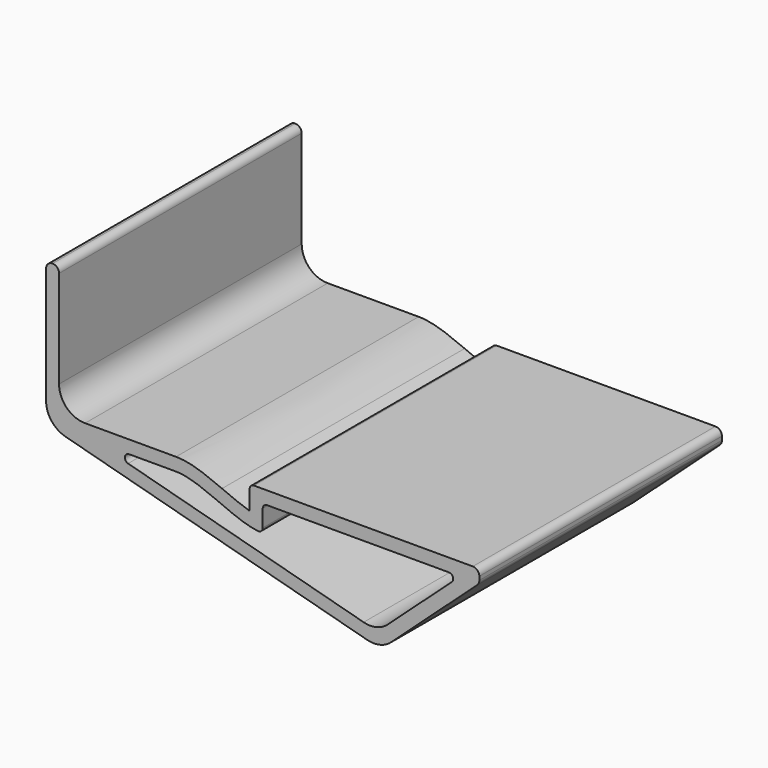
from build123d import *

# Parameters (mm, degrees)
F0_W         = 1.5
F0_H         = 15
F0_H_2       = 1.5
F1_DEPTH     = 35
F2_R         = 3
F3_R         = 0.5
F4_R         = 0.74999
F5_TEXT_SIZE = 7.8123211902
F6_DEPTH     = 0.4


# Not quite as in the source:
# - a fillet or chamfer is up to 0.001 mm smaller than in the source, because OpenCascade refuses the exact size
# - ends of sketch curves that miss each other by under 0.0002 mm in the source are joined
# - Text() gives the source's letters only with a copy of the font that has no kerning and outlines rounded to 1/6400 em; it was checked with that copy


with BuildPart() as f1:
    # F0 (on Front) → F1 (new body)
    with BuildSketch(Plane.XZ):
        with Locations((0.75, 9)):
            Rectangle(F0_W, F0_H)
        with BuildLine():
            Line((1.5, 1.5), (0, 1.5))
            Line((0, 1.5), (0, 0))
            Line((0, 0), (5.7955549577, 0))
            Line((5.7955549577, 0), (15, 0))
            Line((15, 0), (20.3076726165, 0))
            add(Edge.make_bspline(
                [(20.3076726165, 0), (19.9613391426, 0.1480763703), (19.1624921639, 0.4865686334), (17.8864112021, 0.9748848409), (16.4769611274, 1.3772161031), (15.5, 1.5), (15, 1.5)],
                knots=[0.5268596167, 0.5268596167, 0.5268596167, 0.5268596167, 0.625, 0.75, 0.875, 1, 1, 1, 1], degree=3))
            Line((15, 1.5), (1.5, 1.5))
        make_face()
        with BuildLine():
            add(Edge.make_bspline(
                [(23.5000271172, -1.2432669014), (23.3597225948, -1.2025116169), (22.8440957766, -1.0410149339), (21.8859439585, -0.6761057841), (20.9362434779, -0.2693177997), (20.4024591259, -0.0405263808), (20.3076726165, 0)],
                knots=[0.2014712136, 0.2014712136, 0.2014712136, 0.2014712136, 0.25, 0.375, 0.5, 0.5268596167, 0.5268596167, 0.5268596167, 0.5268596167], degree=3))
            Line((20.3076726165, 0), (15, 0))
            add(Edge.make_bspline(
                [(25, -3), (22, -3), (18, 0), (15, 0)],
                knots=[0, 0, 0, 0, 10.4403065089, 10.4403065089, 10.4403065089, 10.4403065089], degree=3))
            Line((25, -3), (25, 0))
            Line((25, 0), (23.5, 0))
            Line((23.5, 0), (23.5000271172, -1.2432669014))
        make_face()
        with Locations((24.25, 0.75)):
            Rectangle(F0_W, F0_H_2)
        Polygon((47.7727761903, 0), (50, 0), (50, 1.5), (25, 1.5), (25, 0), align=None)
        Polygon((39.0252616192, -8.9038730647), (38.6370330516, -10.3527618041), (50, 0), (47.7727761903, 0), (38.2330606413, -8.6916034524), align=None)
        Polygon((5.7955549577, 0), (0, 0), (38.6370330516, -10.3527618041), (39.0252616192, -8.9038730647), (38.2330606413, -8.6916034524), align=None)
    extrude(amount=F1_DEPTH)

    # F2
    f2_edges = [f1.edges().sort_by_distance(p)[0] for p in [
        (1.5, -17.5, 1.5),
        (0, -17.5, 0),
        (38.637033, -17.5, -10.352762),
        (38.233061, -17.5, -8.691603),
    ]]
    fillet(f2_edges, radius=F2_R)

    # F3
    f3_edges = [f1.edges().sort_by_distance(p)[0] for p in [
        (47.772776, -17.5, 0),
        (5.795555, -17.5, 0),
        (15, -17.5, 0),
        (23.5, -17.5, 1.5),
        (25, -17.5, 0),
        (25, -17.5, -3),
    ]]
    fillet(f3_edges, radius=F3_R)

    # F4 (radius 0.75 in the source; OpenCascade refuses exactly that, so slightly less here)
    f4_edges = [f1.edges().sort_by_distance(p)[0] for p in [
        (50, -17.5, 0),
        (50, -17.5, 1.5),
        (1.5, -17.5, 16.5),
        (0, -17.5, 16.5),
    ]]
    fillet(f4_edges, radius=F4_R)

    # F5 (on face) → F6 (cut)
    with BuildSketch(Plane(origin=(0, 0, 0), x_dir=(0.9659258263, 0, -0.2588190451), z_dir=(-0.2588190451, 0, -0.9659258263))):
        with Locations((4.3308436794, 14.6875643715)):
            Text('AIRSTER', F5_TEXT_SIZE, font='Open Sans', font_style=FontStyle.BOLD, text_align=(TextAlign.LEFT, TextAlign.BOTTOM))
    extrude(amount=-F6_DEPTH, mode=Mode.SUBTRACT)


solid = f1.part
